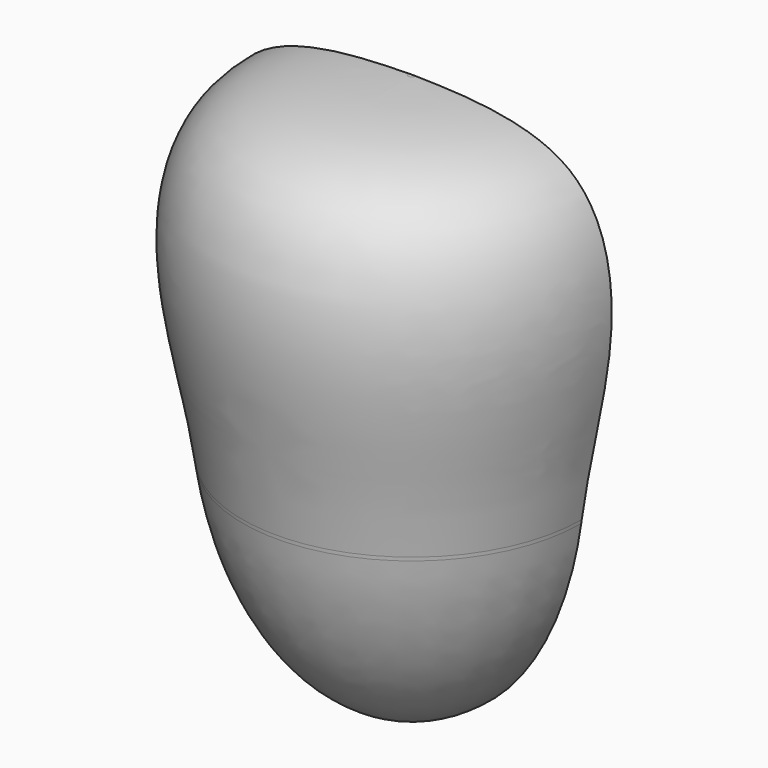
from build123d import *

# Parameters (mm, degrees)
F1_ANGLE = 180
F3_ANGLE = 180


with BuildPart() as f1:
    # F0 (on Front) → F1 (revolve)
    with BuildSketch(Plane.XZ):
        with BuildLine():
            Line((0, 80), (0, -80))
            add(Edge.make_bspline(
                [(0, -80), (50, -80), (50, 0), (50, 80), (0, 80)],
                knots=[3.1415926536, 3.1415926536, 3.1415926536, 4.7123889804, 4.7123889804, 6.2831853072, 6.2831853072, 6.2831853072], degree=2, weights=[1, 0.7071067812, 1, 0.7071067812, 1]))
        make_face()
    revolve(axis=Axis((0, 0, 0), (0, 0, -1)), revolution_arc=F1_ANGLE)

    # F2 (on Front) → F3 (revolve)
    with BuildSketch(Plane.XZ):
        with BuildLine():
            add(Edge.make_bspline(
                [(-48.8691344885, -16.9182652042), (-48.7987705621, -17.4385832037), (-48.7240850007, -17.9573568365)],
                knots=[1.783883564, 1.783883564, 1.783883564, 1.7971923305, 1.7971923305, 1.7971923305], degree=2, weights=[1, 0.9999778597, 1]))
            add(Edge.make_bspline(
                [(-48.7240850007, -17.9573568365), (-48.7716070362, -17.6101579438), (-48.8199705199, -17.2637980693), (-48.8691344885, -16.9182652042)],
                knots=[0, 0, 0, 0, 0.0062919262, 0.0062919262, 0.0062919262, 0.0062919262], degree=3))
        make_face()
        with BuildLine():
            add(Edge.make_bspline(
                [(-48.7240850007, -17.9573568365), (-48.7716070362, -17.6101579438), (-48.8199705199, -17.2637980693), (-48.8691344885, -16.9182652042)],
                knots=[0, 0, 0, 0, 0.0062919262, 0.0062919262, 0.0062919262, 0.0062919262], degree=3))
            add(Edge.make_bspline(
                [(-48.7240850007, -17.9573568365), (-39.7920781648, -80), (0, -80)],
                knots=[1.7971923305, 1.7971923305, 1.7971923305, 3.1415926536, 3.1415926536, 3.1415926536], degree=2, weights=[1, 0.7824535004, 1]))
            Line((0, -80), (0, 80))
            add(Edge.make_bspline(
                [(-1.108818783, 79.9803259153), (-0.7342012018, 79.9871031051), (-0.3644851316, 79.9936072588), (0, 80)],
                knots=[0.9907691128, 0.9907691128, 0.9907691128, 0.9907691128, 1, 1, 1, 1], degree=3))
            add(Edge.make_bspline(
                [(-48.8691344885, -16.9182652042), (-51.690056449, 2.9076616941), (-61.6964555806, 34.2736191316), (-51.0571402446, 78.6418106223), (-14.1928285059, 79.7436236842), (-1.108818783, 79.9803259153)],
                knots=[0.0062919262, 0.0062919262, 0.0062919262, 0.0062919262, 0.3673090138, 0.6683682859, 0.9907691128, 0.9907691128, 0.9907691128, 0.9907691128], degree=3))
        make_face()
        with BuildLine():
            add(Edge.make_bspline(
                [(0, 80), (-0.5544775717, 80), (-1.108818783, 79.9803259153)],
                knots=[0, 0, 0, 0.0221781938, 0.0221781938, 0.0221781938], degree=2, weights=[1, 0.9999385166, 1]))
            add(Edge.make_bspline(
                [(-1.108818783, 79.9803259153), (-0.7342012018, 79.9871031051), (-0.3644851316, 79.9936072588), (0, 80)],
                knots=[0.9907691128, 0.9907691128, 0.9907691128, 0.9907691128, 1, 1, 1, 1], degree=3))
        make_face()
    revolve(axis=Axis((0, 0, 0), (0, 0, 1)), revolution_arc=F3_ANGLE)


solid = f1.part
